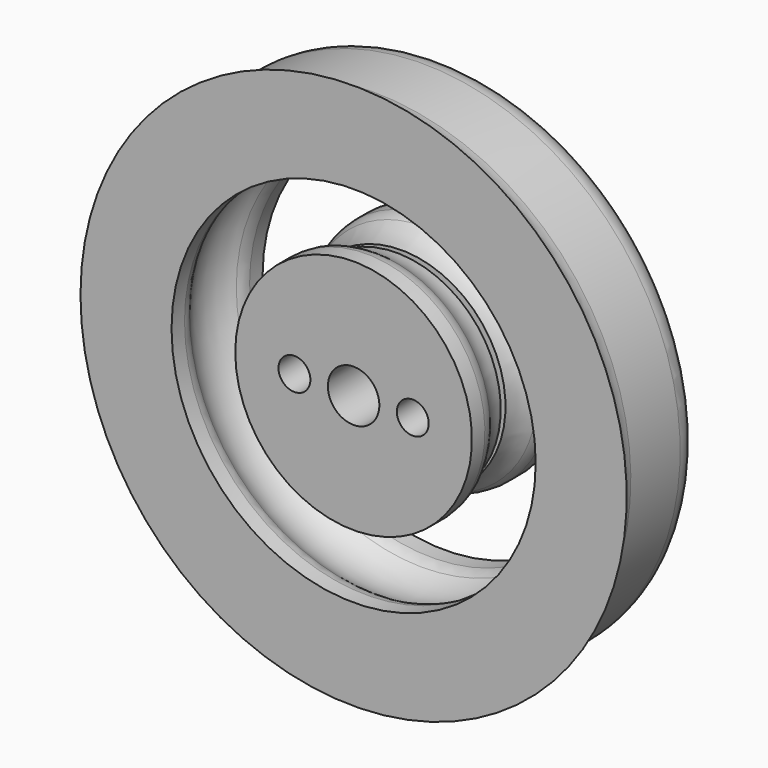
from build123d import *

# Parameters (mm, degrees)
F3_R     = 1.75
F4_DEPTH = 25
F5_DEPTH = 25
F6_R     = 3
F7_R     = 2
F7_2_R   = 2
F7_3_R   = 2
F8_R     = 12.5
F8_R_2   = 11.4125
F8_R_3   = 1.75
F8_R_4   = 4
F9_DEPTH = 0.325


with BuildPart() as f1:
    # F0 (on Top) → F1 (revolve)
    with BuildSketch(Plane.XY):
        with BuildLine():
            Line((-30, 0), (-20, 0))
            Line((-20, 0), (-20, 2.5577572872))
            ThreePointArc((-20, 2.5577572872), (-21.5875, 6.25), (-20, 9.9422427128))
            Line((-20, 9.9422427128), (-20, 12.5))
            Line((-20, 12.5), (-28.2679491924, 12.5))
            Line((-28.2679491924, 12.5), (-28.2679491924, 1))
            Line((-28.2679491924, 1), (-30, 0))
        make_face()
    revolve(axis=Axis((0, 6.25, 0), (0, 1, 0)))

    # F6
    f6_edges = [f1.edges().sort_by_distance(p)[0] for p in [
        (28.267949, 1, 0),
        (28.267949, 12.5, 0),
    ]]
    fillet(f6_edges, radius=F6_R)

    # F7
    f7_edges = [f1.edges().sort_by_distance(p)[0] for p in [
        (20, 2.557757, 0),
        (20, 9.942243, 0),
    ]]
    fillet(f7_edges, radius=F7_R)


with BuildPart() as f1b:
    # F0 (on Top) → F1, piece 2 (revolve)
    with BuildSketch(Plane.XY):
        with BuildLine():
            Line((-4, 6.25), (-4, 12.5))
            Line((-4, 12.5), (-13, 12.5))
            Line((-13, 12.5), (-13, 9.9422427128))
            ThreePointArc((-13, 9.9422427128), (-11.8261950057, 8.2595280851), (-11.4125, 6.25))
            Line((-11.4125, 6.25), (-4, 6.25))
        make_face()
    revolve(axis=Axis((0, 6.25, 0), (0, 1, 0)))


with BuildPart() as f2:
    # F0 (on Top) → F2 (revolve)
    with BuildSketch(Plane.XY):
        with BuildLine():
            Line((-13, 0), (-2.825, 0))
            Line((-2.825, 0), (-2.825, 12.5))
            Line((-2.825, 12.5), (-4, 12.5))
            Line((-4, 12.5), (-4, 6.25))
            Line((-4, 6.25), (-11.4125, 6.25))
            ThreePointArc((-11.4125, 6.25), (-11.8261950057, 4.2404719149), (-13, 2.5577572872))
            Line((-13, 2.5577572872), (-13, 0))
        make_face()
    revolve(axis=Axis((0, 6.25, 0), (0, 1, 0)))


with BuildPart() as f4_tool:
    # F3 (on face) → F4 (new body)
    with BuildSketch(Plane(origin=(0, 12.5, 0), x_dir=(-1, 0, 0), z_dir=(0, 1, 0))):
        with Locations((-6.5, 0)):
            Circle(F3_R)
        with BuildLine():
            ThreePointArc((8.25, 0), (6.5, 1.75), (4.75, 0))
            ThreePointArc((4.75, 0), (6.5, -1.75), (8.25, 0))
        make_face()
    extrude(amount=-F4_DEPTH)


with BuildPart() as f1b_1:
    add(f1b.part)

    # F4: cut by f4_tool
    add(f4_tool.part, mode=Mode.SUBTRACT)

    # F3 (on face) → F5 (cut)
    with BuildSketch(Plane(origin=(0, 12.5, 0), x_dir=(-1, 0, 0), z_dir=(0, 1, 0))):
        with BuildLine():
            ThreePointArc((4, 0), (0, -4), (-4, 0))
            Line((-4, 0), (-4.325, 0))
            ThreePointArc((-4.325, 0), (0, -4.325), (4.325, 0))
            Line((4.325, 0), (4, 0))
        make_face()
        with BuildLine():
            Line((-4.325, 0), (-4, 0))
            ThreePointArc((-4, 0), (0, 4), (4, 0))
            Line((4, 0), (4.325, 0))
            ThreePointArc((4.325, 0), (0, 4.325), (-4.325, 0))
        make_face()
    extrude(amount=-F5_DEPTH, mode=Mode.SUBTRACT)

    # F7#2
    f7_2_edges = [f1b_1.edges().sort_by_distance(p)[0] for p in [
        (13, 9.942243, 0),
    ]]
    fillet(f7_2_edges, radius=F7_2_R)


with BuildPart() as f2_1:
    add(f2.part)

    # F4: cut by f4_tool
    add(f4_tool.part, mode=Mode.SUBTRACT)

    # F7#3
    f7_3_edges = [f2_1.edges().sort_by_distance(p)[0] for p in [
        (13, 2.557757, 0),
    ]]
    fillet(f7_3_edges, radius=F7_3_R)


with BuildPart() as f9_tool:
    # F8 (on face) → F9 (new body, symmetric)
    with BuildSketch(Plane(origin=(0, 6.25, 0), x_dir=(-1, 0, 0), z_dir=(0, 1, 0))):
        Circle(F8_R)
        Circle(F8_R_2, mode=Mode.SUBTRACT)
        Circle(F8_R_2)
        with Locations((-6.5, 0)):
            Circle(F8_R_3, mode=Mode.SUBTRACT)
        Circle(F8_R_4, mode=Mode.SUBTRACT)
        with Locations((6.5, 0)):
            Circle(F8_R_3, mode=Mode.SUBTRACT)
    extrude(amount=F9_DEPTH, both=True)


with BuildPart() as f1b_2:
    add(f1b_1.part)

    # F9: cut by f9_tool
    add(f9_tool.part, mode=Mode.SUBTRACT)


with BuildPart() as f2_2:
    add(f2_1.part)

    # F9: cut by f9_tool
    add(f9_tool.part, mode=Mode.SUBTRACT)


solid = Compound([f1.part, f1b_2.part, f2_2.part])
